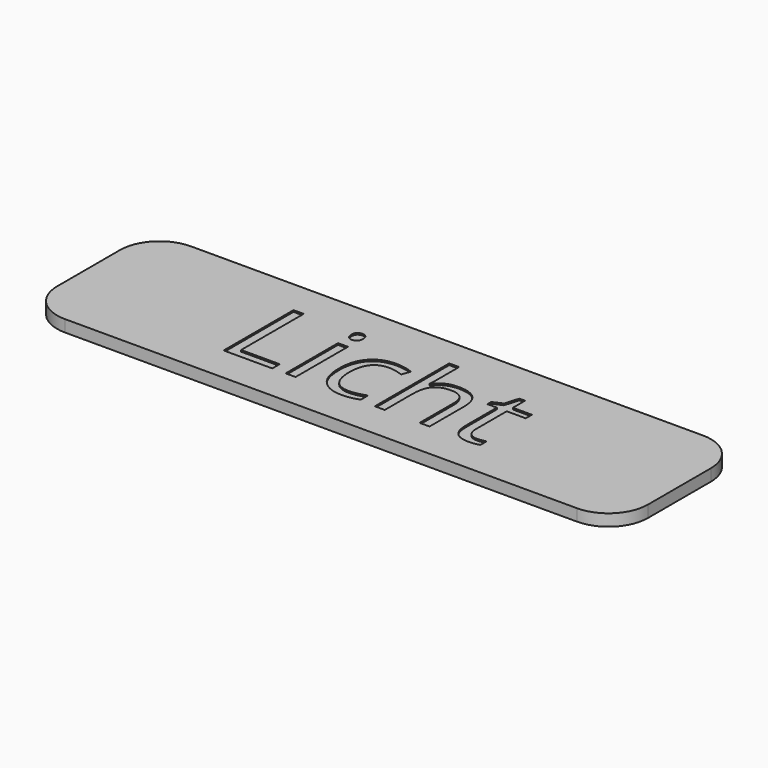
from build123d import *

# Parameters (mm, degrees)
F1_DEPTH     = 1.5
F2_TEXT_SIZE = 15.527301649
F3_DEPTH     = 0.2


# Not quite as in the source:
# - Text() gives the source's letters only with a copy of the font that has no kerning and outlines rounded to 1/6400 em; it was checked with that copy


with BuildPart() as f1:
    # F0 (on Top) → F1 (new body)
    with BuildSketch(Plane.XY):
        with BuildLine():
            ThreePointArc((37.5, 5), (36.0355339059, 8.5355339059), (32.5, 10))
            Line((32.5, 10), (-32.5, 10))
            ThreePointArc((-32.5, 10), (-36.0355339059, 8.5355339059), (-37.5, 5))
            Line((-37.5, 5), (-37.5, -5))
            ThreePointArc((-37.5, -5), (-36.0355339059, -8.5355339059), (-32.5, -10))
            Line((-32.5, -10), (32.5, -10))
            ThreePointArc((32.5, -10), (36.0355339059, -8.5355339059), (37.5, -5))
            Line((37.5, -5), (37.5, 5))
        make_face()
    extrude(amount=F1_DEPTH)

    # F2 (on face) → F3 (cut)
    with BuildSketch(Plane.XY.offset(1.5)):
        with Locations((-17.5361462999, -5.4303565994)):
            Text('Licht', F2_TEXT_SIZE, font='Open Sans', text_align=(TextAlign.LEFT, TextAlign.BOTTOM))
    extrude(amount=-F3_DEPTH, mode=Mode.SUBTRACT)


solid = f1.part
